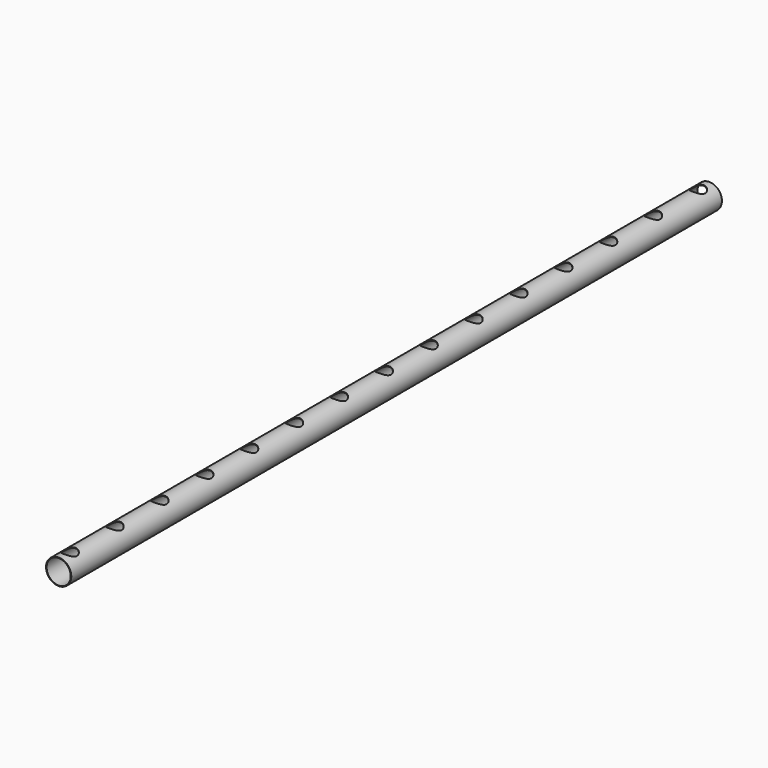
from build123d import *

# Parameters (mm, degrees)
F0_R     = 45
F0_R_2   = 43
F1_DEPTH = 1450
F4_D     = 50
F4_DEPTH = 50
F4_TIP   = 15.0215154757


# Not quite as in the source:
# - a feature names something its author has since deleted; it is built from what else it names


with BuildPart() as f1:
    # F0 (on Front) → F1 (new body, symmetric)
    with BuildSketch(Plane.XZ):
        Circle(F0_R)
        Circle(F0_R_2, mode=Mode.SUBTRACT)
    extrude(amount=F1_DEPTH, both=True)

    # F4
    with Locations(Plane.XY.offset(45)):
        with Locations((0, -1400), (0, -1200), (0, -1000), (0, -800), (0, -600), (0, -400), (0, -200), (0, 0), (0, 200), (0, 400), (0, 600), (0, 800), (0, 1000), (0, 1200), (0, 1400)):
            Hole(F4_D / 2, depth=F4_DEPTH)
            with Locations((0, 0, -(F4_DEPTH + F4_TIP / 2))):  # 118° drill point
                Cone(0, F4_D / 2, F4_TIP, mode=Mode.SUBTRACT)


solid = f1.part
